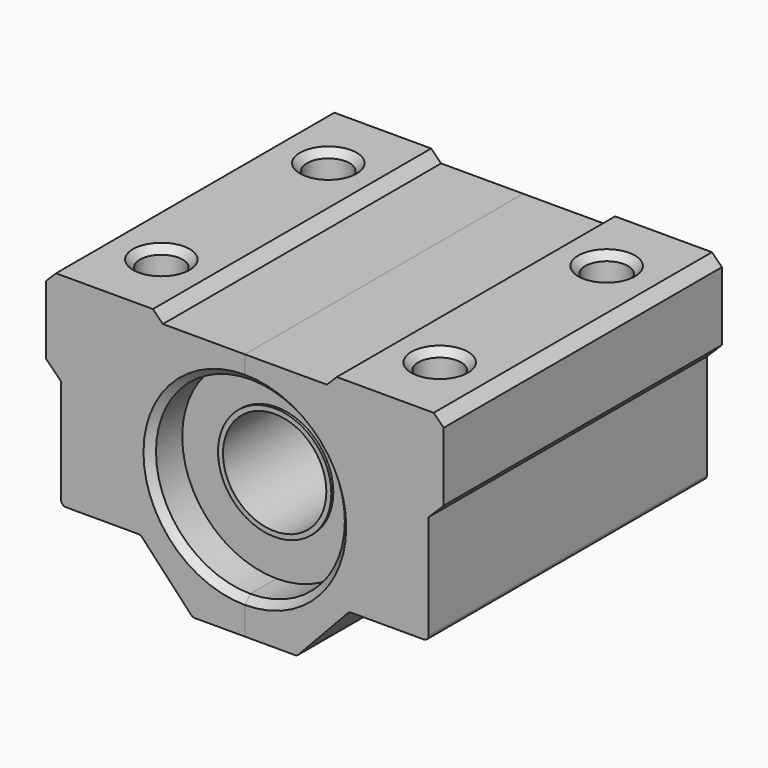
from build123d import *
from build123d import SkipClean  # not in build123d's __all__

# Parameters (mm, degrees)
F1_DEPTH       = 17.5
F2_SIZE        = 0.99999
F3_SIZE        = 1.49999
F4_R           = 0.5
F6_D           = 4
F6_CBORE_D     = 4.3
F6_CBORE_DEPTH = 12
F7_SIZE        = 0.7
F0_R           = 5.7
F8_DEPTH       = 13.5
F0_R_2         = 5.2
F9_DEPTH       = 13.75


# Not quite as in the source:
# - a fillet or chamfer is up to 0.001 mm smaller than in the source, because OpenCascade refuses the exact size


with BuildPart() as f1:
    # F0 (on Front) → F1 (new body, symmetric)
    with BuildSketch(Plane.XZ):
        with BuildLine():
            ThreePointArc((0, 9.5), (6.7175144213, 6.7175144213), (9.5, 0))
            ThreePointArc((9.5, 0), (6.7175144213, -6.7175144213), (0, -9.5))
            Line((0, -9.5), (0, -13))
            Line((0, -13), (5.25, -13))
            Line((5.25, -13), (10.5, -7.4))
            Line((10.5, -7.4), (18.5, -7.4))
            Line((18.5, -7.4), (18.5, 3.6))
            Line((18.5, 3.6), (20, 3.6))
            Line((20, 3.6), (20, 13))
            Line((20, 13), (9.25, 13))
            Line((9.25, 13), (9.25, 12))
            Line((9.25, 12), (0, 12))
            Line((0, 12), (0, 9.5))
        make_face()
    extrude(amount=F1_DEPTH, both=True)

    # F2 (size 1 in the source; OpenCascade refuses exactly that, so slightly less here)
    f2_edges = [f1.edges().sort_by_distance(p)[0] for p in [
        (9.25, 0, 12),
        (20, 0, 13),
    ]]
    chamfer(f2_edges, length=F2_SIZE)

    # F3 (size 1.5 in the source; OpenCascade refuses exactly that, so slightly less here)
    f3_edges = [f1.edges().sort_by_distance(p)[0] for p in [
        (20, 0, 3.6),
    ]]
    chamfer(f3_edges, length=F3_SIZE)

    # F4
    f4_edges = [f1.edges().sort_by_distance(p)[0] for p in [
        (18.5, 0, -7.4),
        (10.5, 0, -7.4),
        (5.25, 0, -13),
    ]]
    fillet(f4_edges, radius=F4_R)

    # F6 (through all)
    with Locations(Plane.XY.offset(13)):
        with Locations((14, 10.5), (14, -10.5)):
            CounterBoreHole(F6_D / 2, F6_CBORE_D / 2, F6_CBORE_DEPTH)

    # F7
    f7_edges = [f1.edges().sort_by_distance(p)[0] for p in [
        (9.5, -17.5, 0),
        (9.5, 17.5, 0),
        (11.85, 10.5, 13),
        (11.85, -10.5, 13),
    ]]
    chamfer(f7_edges, length=F7_SIZE)

    # F10: F1 across plane


with BuildPart() as f8:
    # F0 (on Front) → F8 (new body, symmetric)
    with BuildSketch(Plane.XZ):
        with BuildLine():
            ThreePointArc((0, -9.5), (6.7175144213, -6.7175144213), (9.5, 0))
            ThreePointArc((9.5, 0), (6.7175144213, 6.7175144213), (0, 9.5))
            ThreePointArc((0, 9.5), (-9.5, 0), (0, -9.5))
        make_face()
        Circle(F0_R, mode=Mode.SUBTRACT)
    extrude(amount=F8_DEPTH, both=True)

    # F0 (on Front) → F9 (join, symmetric)
    with BuildSketch(Plane.XZ):
        Circle(F0_R)
        Circle(F0_R_2, mode=Mode.SUBTRACT)
    extrude(amount=F9_DEPTH, both=True)


with BuildPart() as f1_1:
    add(f1.part, clean=False)
    with SkipClean():  # cleaning this boolean's faces spoils the solid; the shape is the same uncleaned
        add(f1.part.mirror(Plane.YZ), clean=False)


solid = Compound([f8.part, f1_1.part])
